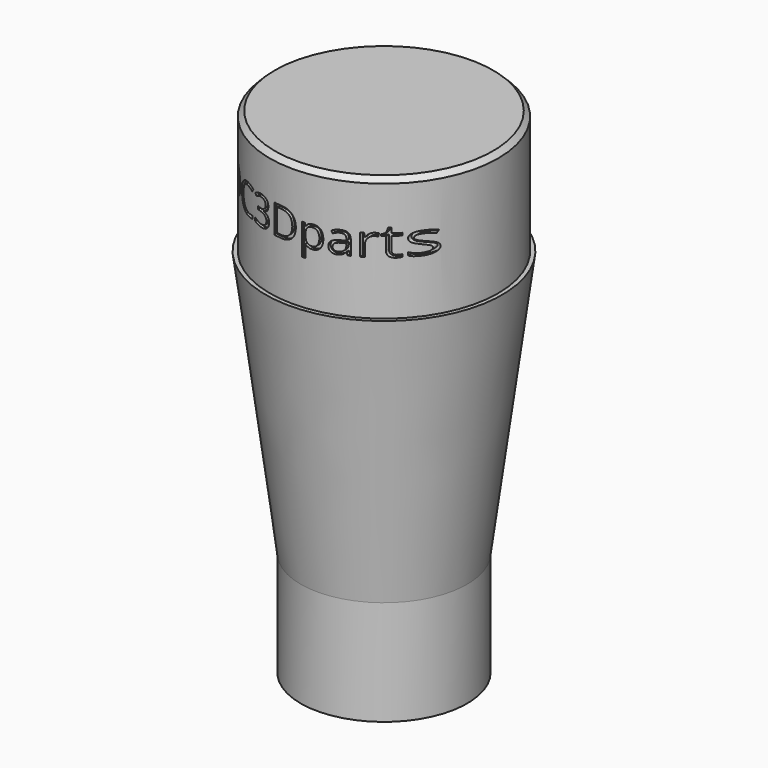
from build123d import *

# Parameters (mm, degrees)
F2_SIZE      = 1.2
F4_TEXT_SIZE = 9.7222222222
F5_DEPTH     = 40
F6_W         = 27
F6_H         = 32.5915426314


# Not quite as in the source:
# - Text() gives the source's letters only with a copy of the font that has no kerning and outlines rounded to 1/6400 em; it was checked with that copy


with BuildPart() as f1:
    # F0 (on Front) → F1 (revolve)
    with BuildSketch(Plane.XZ):
        Polygon((0, 73.2666279856), (-27.685, 73.2666279856), (-27.685, 43.2666279856), (-28.685, 43.2666279856), (-20.2, -21.2990029593), (-20.2, -46.7333720144), (0, -46.7333720144), align=None)
    revolve(axis=Axis((0, 0, -2.5966958965), (0, 0, -1)))

    # F2
    f2_edges = [f1.edges().sort_by_distance(p)[0] for p in [
        (27.685, 0, 73.266628),
    ]]
    chamfer(f2_edges, length=F2_SIZE)


with BuildPart() as f5:
    # F4 (on offset) → F5 (new body, through all)
    with BuildSketch(Plane.XZ.offset(40)):
        with Locations((-24.512081203, 56.2920023986)):
            Text('DC3Dparts', F4_TEXT_SIZE, font='Open Sans', text_align=(TextAlign.LEFT, TextAlign.BOTTOM))
    extrude(amount=-F5_DEPTH)


with BuildPart() as f7:
    # F6 (on Front) → F7 (revolve)
    with BuildSketch(Plane.XZ):
        with Locations((-13.5, 65.4938702357)):
            Rectangle(F6_W, F6_H)
    revolve(axis=Axis((0, 0, 65.4938702357), (0, 0, 1)))


with BuildPart() as f5_1:
    add(f5.part)

    # F8: cut F7
    add(f7.part, mode=Mode.SUBTRACT)


with BuildPart() as f1_1:
    add(f1.part)

    # F9: cut F5
    add(f5_1.part, mode=Mode.SUBTRACT)


solid = f1_1.part
